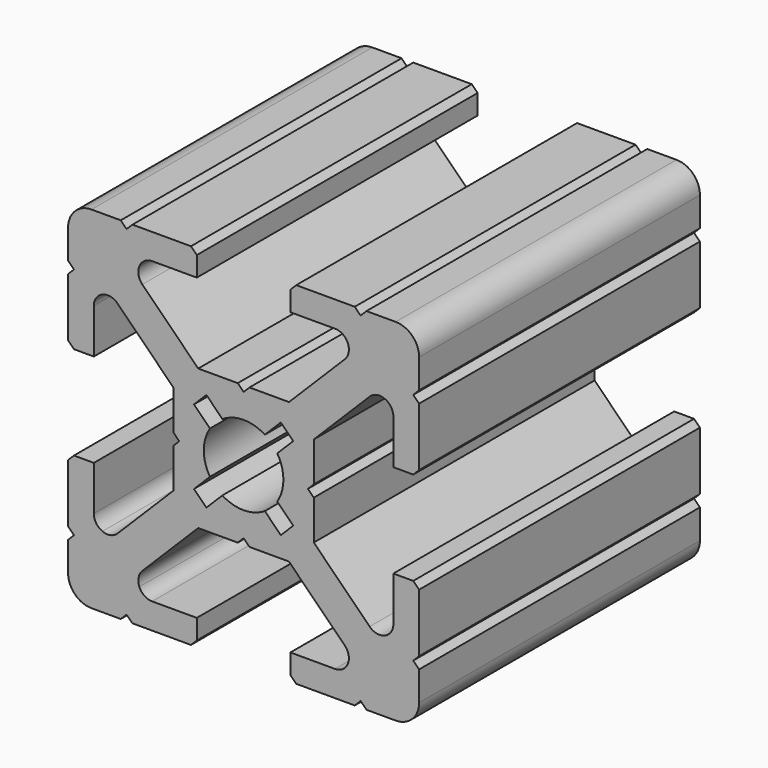
from build123d import *

# Parameters (mm, degrees)
F1_DEPTH = 30


# Not quite as in the source:
# - ends of sketch curves that miss each other by under 0.0002 mm in the source are joined


with BuildPart() as f1:
    # F0 (on Front) → F1 (new body)
    with BuildSketch(Plane.XZ):
        with BuildLine():
            ThreePointArc((-12.0672760652, 8.9096491574), (-11.3814883912, 8.9771930389), (-10.7737513132, 8.6523506868))
            Line((-10.7737513132, 8.6523506868), (-6, 3.8786))
            Line((-6, 3.8786), (-6, 0.5))
            Line((-6, 0.5), (-5.5, 0))
            Line((-5.5, 0), (-6, -0.5))
            Line((-6, -0.5), (-6, -3.8786))
            Line((-6, -3.8786), (-10.7738, -8.6524))
            ThreePointArc((-10.7738, -8.6524), (-11.3814883912, -8.9771930389), (-12.0672760652, -8.9096491574))
            ThreePointArc((-12.0672760652, -8.9096491574), (-12.5999492171, -8.4725051968), (-12.799999999, -7.8131))
            Line((-12.799999999, -7.8131), (-12.8, -4))
            Line((-12.8, -4), (-14.5, -4))
            Line((-14.5, -4), (-15, -4.5))
            Line((-15, -4.5), (-15, -9.5))
            Line((-15, -9.5), (-14.5, -10))
            Line((-14.5, -10), (-15, -10.5))
            Line((-15, -10.5), (-15, -13))
            ThreePointArc((-15, -13), (-14.4141844722, -14.4142216524), (-13, -15.0000239995))
            Line((-13, -15.0000239995), (-10.5, -15))
            Line((-10.5, -15), (-10, -14.5))
            Line((-10, -14.5), (-9.5, -15))
            Line((-9.5, -15), (-4.5, -15))
            Line((-4.5, -15), (-4, -14.5))
            Line((-4, -14.5), (-4, -12.8))
            Line((-4, -12.8), (-7.8131, -12.8))
            ThreePointArc((-7.8131, -12.8), (-8.4725048128, -12.5999494737), (-8.9096488038, -12.0672769187))
            ThreePointArc((-8.9096488038, -12.0672769187), (-8.977199798, -11.3815223738), (-8.6523996854, -10.7738003146))
            Line((-8.6523996854, -10.7738003146), (-3.8786, -6))
            Line((-3.8786, -6), (-0.5, -6))
            Line((-0.5, -6), (0, -5.5))
            Line((0, -5.5), (0.5, -6))
            Line((0.5, -6), (3.8786, -6))
            Line((3.8786, -6), (8.6524, -10.7738))
            ThreePointArc((8.6524, -10.7738), (8.977199798, -11.3815223738), (8.9096491574, -12.0672760652))
            ThreePointArc((8.9096491574, -12.0672760652), (8.4725048128, -12.5999494737), (7.8131, -12.799999999))
            Line((7.8131, -12.799999999), (4, -12.8))
            Line((4, -12.8), (4, -14.5))
            Line((4, -14.5), (4.5, -15))
            Line((4.5, -15), (9.5, -15))
            Line((9.5, -15), (10, -14.5))
            Line((10, -14.5), (10.5, -15))
            Line((10.5, -15), (13, -15))
            ThreePointArc((13, -15), (14.4141844722, -14.4142216524), (14.999955, -13.000024))
            Line((14.999955, -13.000024), (15, -10.5))
            Line((15, -10.5), (14.5, -10))
            Line((14.5, -10), (15, -9.5))
            Line((15, -9.5), (15, -4.5))
            Line((15, -4.5), (14.5, -4))
            Line((14.5, -4), (12.8, -4))
            Line((12.8, -4), (12.8, -7.8131))
            ThreePointArc((12.8, -7.8131), (12.5999492171, -8.4725051968), (12.0672760652, -8.9096491574))
            ThreePointArc((12.0672760652, -8.9096491574), (11.3814883912, -8.9771930389), (10.7737513132, -8.6523506868))
            Line((10.7737513132, -8.6523506868), (6, -3.8786))
            Line((6, -3.8786), (6, -0.5))
            Line((6, -0.5), (5.5, 0))
            Line((5.5, 0), (6, 0.5))
            Line((6, 0.5), (6, 3.8786))
            Line((6, 3.8786), (10.7738, 8.6524))
            ThreePointArc((10.7738, 8.6524), (11.3814883912, 8.9771930389), (12.0672760652, 8.9096491574))
            ThreePointArc((12.0672760652, 8.9096491574), (12.5999492171, 8.4725051968), (12.799999999, 7.8131))
            Line((12.799999999, 7.8131), (12.8, 4))
            Line((12.8, 4), (14.5, 4))
            Line((14.5, 4), (15, 4.5))
            Line((15, 4.5), (15, 9.5))
            Line((15, 9.5), (14.5, 10))
            Line((14.5, 10), (15, 10.5))
            Line((15, 10.5), (15, 13))
            ThreePointArc((15, 13), (14.4141844722, 14.4142216524), (13, 15.0000239995))
            Line((13, 15.0000239995), (10.5, 15))
            Line((10.5, 15), (10, 14.5))
            Line((10, 14.5), (9.5, 15))
            Line((9.5, 15), (4.5, 15))
            Line((4.5, 15), (4, 14.5))
            Line((4, 14.5), (4, 12.8))
            Line((4, 12.8), (7.8131, 12.8))
            ThreePointArc((7.8131, 12.8), (8.4725048128, 12.5999494737), (8.9096488038, 12.0672769187))
            ThreePointArc((8.9096488038, 12.0672769187), (8.977199798, 11.3815223738), (8.6523996854, 10.7738003146))
            Line((8.6523996854, 10.7738003146), (3.8786, 6))
            Line((3.8786, 6), (0.5, 6))
            Line((0.5, 6), (0, 5.5))
            Line((0, 5.5), (-0.5, 6))
            Line((-0.5, 6), (-3.8786, 6))
            Line((-3.8786, 6), (-8.6524, 10.7738))
            ThreePointArc((-8.6524, 10.7738), (-8.977199798, 11.3815223738), (-8.9096491574, 12.0672760652))
            ThreePointArc((-8.9096491574, 12.0672760652), (-8.4725048128, 12.5999494737), (-7.8131, 12.799999999))
            Line((-7.8131, 12.799999999), (-4, 12.8))
            Line((-4, 12.8), (-4, 14.5))
            Line((-4, 14.5), (-4.5, 15))
            Line((-4.5, 15), (-9.5, 15))
            Line((-9.5, 15), (-10, 14.5))
            Line((-10, 14.5), (-10.5, 15))
            Line((-10.5, 15), (-13, 15))
            ThreePointArc((-13, 15), (-14.4141844722, 14.4142216524), (-14.999955, 13.000024))
            Line((-14.999955, 13.000024), (-15, 10.5))
            Line((-15, 10.5), (-14.5, 10))
            Line((-14.5, 10), (-15, 9.5))
            Line((-15, 9.5), (-15, 4.5))
            Line((-15, 4.5), (-14.5, 4))
            Line((-14.5, 4), (-12.8, 4))
            Line((-12.8, 4), (-12.8, 7.8131))
            ThreePointArc((-12.8, 7.8131), (-12.5999492171, 8.4725051968), (-12.0672760652, 8.9096491574))
        make_face()
        with BuildLine():
            Line((-4.2426, -3.182), (-2.8752, -1.8146))
            ThreePointArc((-2.8752, -1.8146), (-3.4, 0), (-2.8752481958, 1.8146481236))
            Line((-2.8752481958, 1.8146481236), (-4.2426, 3.182))
            Line((-4.2426, 3.182), (-3.182, 4.2426))
            Line((-3.182, 4.2426), (-1.8146, 2.8752))
            ThreePointArc((-1.8146, 2.8752), (0, 3.4), (1.8146481236, 2.8752481958))
            Line((1.8146481236, 2.8752481958), (3.182, 4.2426))
            Line((3.182, 4.2426), (4.2426, 3.182))
            Line((4.2426, 3.182), (2.8752, 1.8146))
            ThreePointArc((2.8752, 1.8146), (3.4, 0), (2.8752481958, -1.8146481236))
            Line((2.8752481958, -1.8146481236), (4.2426, -3.182))
            Line((4.2426, -3.182), (3.182, -4.2426))
            Line((3.182, -4.2426), (1.8146, -2.8752))
            ThreePointArc((1.8146, -2.8752), (0, -3.4), (-1.8146481236, -2.8752481958))
            Line((-1.8146481236, -2.8752481958), (-3.182, -4.2426))
            Line((-3.182, -4.2426), (-4.2426, -3.182))
        make_face(mode=Mode.SUBTRACT)
    extrude(amount=F1_DEPTH)


solid = f1.part
